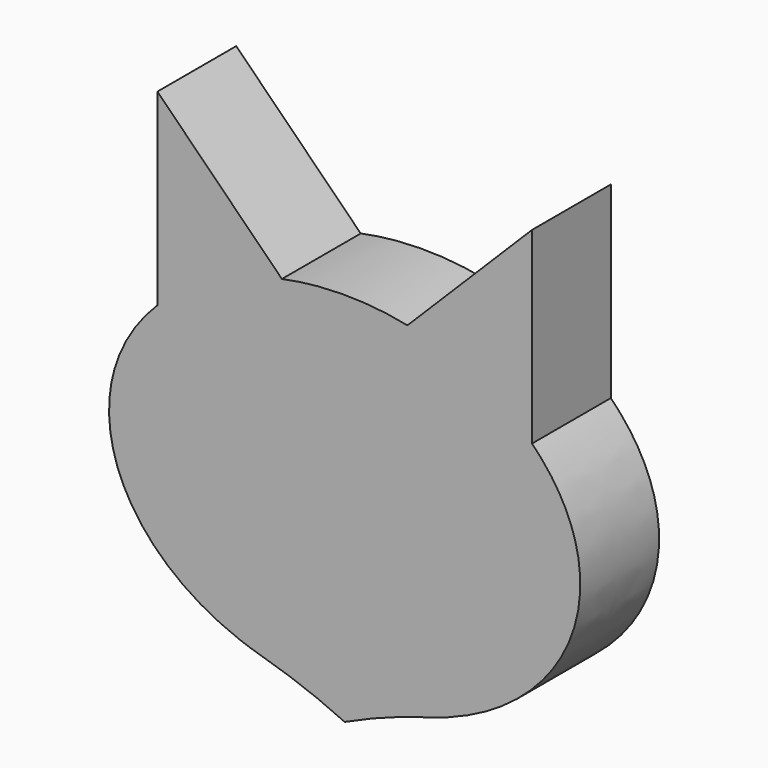
from build123d import *

# Parameters (mm, degrees)
F1_DEPTH    = 25.4
F2_T1_DEPTH = 25.4


# Not quite as in the source:
# - a fillet or chamfer that OpenCascade refuses, or shapes differently, is made with other operations: its cross-section is extruded or revolved along the edge and cut away or added


with BuildPart() as f1:
    # F0 (on Front) → F1 (new body)
    with BuildSketch(Plane.XZ):
        with BuildLine():
            Line((5.7879454147, -45.7212891166), (48.2777159909, 27.8731523232))
            Line((48.2777159909, 27.8731523232), (-48.2777159909, 27.8731523232))
            Line((-48.2777159909, 27.8731523232), (-5.7879454147, -45.7212891166))
            add(Edge.make_bspline(
                [(-5.7879454147, -45.7212891166), (0, -46.1402392948), (5.7879454147, -45.7212891166)],
                knots=[4.6169555149, 4.6169555149, 4.6169555149, 4.8078224459, 4.8078224459, 4.8078224459], degree=2, weights=[1, 0.9954496819, 1]))
        make_face()
        with BuildLine():
            Line((-5.7879454147, -45.7212891166), (-48.2777159909, 27.8731523232))
            add(Edge.make_bspline(
                [(-48.2777159909, 27.8731523232), (-109.7072560683, -32.9641410321), (-9.810773421, -45.327213485)],
                knots=[2.489491462, 2.489491462, 2.489491462, 4.5501606403, 4.5501606403, 4.5501606403], degree=2, weights=[1, 0.5145319732, 1]))
            add(Edge.make_bspline(
                [(-9.810773421, -45.327213485), (-7.808065209, -45.575066323), (-5.7879454147, -45.7212891166)],
                knots=[4.5501606403, 4.5501606403, 4.5501606403, 4.6169555149, 4.6169555149, 4.6169555149], degree=2, weights=[1, 0.9994423574, 1]))
        make_face()
        with BuildLine():
            Line((-48.2777159909, 27.8731523232), (48.2777159909, 27.8731523232))
            add(Edge.make_bspline(
                [(48.2777159909, 27.8731523232), (35.8781903029, 40.1531332703), (16.1845055423, 44.2698445856)],
                knots=[0.6521011916, 0.6521011916, 0.6521011916, 1.3010879793, 1.3010879793, 1.3010879793], degree=2, weights=[1, 0.9478123686, 1]))
            add(Edge.make_bspline(
                [(16.1845055423, 44.2698445856), (0, 47.6530071531), (-16.1845055423, 44.2698445856)],
                knots=[1.3010879793, 1.3010879793, 1.3010879793, 1.8405046743, 1.8405046743, 1.8405046743], degree=2, weights=[1, 0.9638486483, 1]))
            add(Edge.make_bspline(
                [(-16.1845055423, 44.2698445856), (-35.8781903029, 40.1531332703), (-48.2777159909, 27.8731523232)],
                knots=[1.8405046743, 1.8405046743, 1.8405046743, 2.489491462, 2.489491462, 2.489491462], degree=2, weights=[1, 0.9478123686, 1]))
        make_face()
        with BuildLine():
            add(Edge.make_bspline(
                [(9.810773421, -45.327213485), (60.741170722, -39.0241267776), (60.741170722, 0)],
                knots=[4.8746173204, 4.8746173204, 4.8746173204, 6.2831853072, 6.2831853072, 6.2831853072], degree=2, weights=[1, 0.762075353, 1]))
            add(Edge.make_bspline(
                [(60.741170722, 0), (60.741170722, 15.5298586774), (48.2777159909, 27.8731523232)],
                knots=[0, 0, 0, 0.6521011916, 0.6521011916, 0.6521011916], degree=2, weights=[1, 0.947314739, 1]))
            Line((48.2777159909, 27.8731523232), (5.7879454147, -45.7212891166))
            add(Edge.make_bspline(
                [(5.7879454147, -45.7212891166), (7.808065209, -45.575066323), (9.810773421, -45.327213485)],
                knots=[4.8078224459, 4.8078224459, 4.8078224459, 4.8746173204, 4.8746173204, 4.8746173204], degree=2, weights=[1, 0.9994423574, 1]))
        make_face()
        with BuildLine():
            add(Edge.make_bspline(
                [(48.2777159909, 27.8731523232), (35.8781903029, 40.1531332703), (16.1845055423, 44.2698445856)],
                knots=[0.6521011916, 0.6521011916, 0.6521011916, 1.3010879793, 1.3010879793, 1.3010879793], degree=2, weights=[1, 0.9478123686, 1]))
            Line((48.2777159909, 27.8731523232), (48.2777159909, 76.3630550342))
            Line((48.2777159909, 76.3630550342), (16.1845055423, 44.2698445856))
        make_face()
        with BuildLine():
            Line((-48.2777159909, 76.3630550342), (-48.2777159909, 27.8731523232))
            add(Edge.make_bspline(
                [(-16.1845055423, 44.2698445856), (-35.8781903029, 40.1531332703), (-48.2777159909, 27.8731523232)],
                knots=[1.8405046743, 1.8405046743, 1.8405046743, 2.489491462, 2.489491462, 2.489491462], degree=2, weights=[1, 0.9478123686, 1]))
            Line((-16.1845055423, 44.2698445856), (-48.2777159909, 76.3630550342))
        make_face()
        with BuildLine():
            Line((4.1178109195, -48.6140469177), (5.7879454147, -45.7212891166))
            add(Edge.make_bspline(
                [(-5.7879454147, -45.7212891166), (0, -46.1402392948), (5.7879454147, -45.7212891166)],
                knots=[4.6169555149, 4.6169555149, 4.6169555149, 4.8078224459, 4.8078224459, 4.8078224459], degree=2, weights=[1, 0.9954496819, 1]))
            Line((-5.7879454147, -45.7212891166), (-4.1178109195, -48.6140469177))
            Line((-4.1178109195, -48.6140469177), (0, -50.9914661606))
            Line((0, -50.9914661606), (4.1178109195, -48.6140469177))
        make_face()
        with BuildLine():
            add(Edge.make_bspline(
                [(-9.810773421, -45.327213485), (-7.808065209, -45.575066323), (-5.7879454147, -45.7212891166)],
                knots=[4.5501606403, 4.5501606403, 4.5501606403, 4.6169555149, 4.6169555149, 4.6169555149], degree=2, weights=[1, 0.9994423574, 1]))
            Line((-9.810773421, -45.327213485), (-4.1178109195, -48.6140469177))
            Line((-4.1178109195, -48.6140469177), (-5.7879454147, -45.7212891166))
        make_face()
        with BuildLine():
            Line((4.1178109195, -48.6140469177), (9.810773421, -45.327213485))
            add(Edge.make_bspline(
                [(5.7879454147, -45.7212891166), (7.808065209, -45.575066323), (9.810773421, -45.327213485)],
                knots=[4.8078224459, 4.8078224459, 4.8078224459, 4.8746173204, 4.8746173204, 4.8746173204], degree=2, weights=[1, 0.9994423574, 1]))
            Line((5.7879454147, -45.7212891166), (4.1178109195, -48.6140469177))
        make_face()
    extrude(amount=F1_DEPTH)

    # F2: fillet of radius 142.6504443884 on 2 edges, made by hand

    # F2_s2 → F2_t1 (join)
    with BuildSketch(Plane.XZ):
        with BuildLine():
            ThreePointArc((-21.4235280397, -42.9786100328), (-10.5509045607, -46.554957102), (0, -50.9914661606))
            Line((0, -50.9914661606), (1.2104831944, -48.40798205))
            ThreePointArc((1.2104831944, -48.40798205), (-3.4788822666, -45.6885616488), (-8.3842689771, -42.856435311))
            Line((-8.3842689771, -42.856435311), (-9.4603616605, -42.4958054763))
            ThreePointArc((-9.4603616605, -42.4958054763), (-15.0980189089, -41.5804647318), (-20.6415154061, -40.2348687996))
            Line((-20.6415154061, -40.2348687996), (-21.4235280397, -42.9786100328))
        make_face()
        with BuildLine():
            ThreePointArc((0, -50.9914661606), (10.5509045607, -46.554957102), (21.4235280397, -42.9786100328))
            Line((21.4235280397, -42.9786100328), (20.6415154061, -40.2348687996))
            ThreePointArc((20.6415154061, -40.2348687996), (15.0980189089, -41.5804647318), (9.4603616605, -42.4958054763))
            Line((9.4603616605, -42.4958054763), (8.3842689771, -42.856435311))
            ThreePointArc((8.3842689771, -42.856435311), (3.4788822666, -45.6885616488), (-1.2104831944, -48.40798205))
            Line((-1.2104831944, -48.40798205), (0, -50.9914661606))
        make_face()
    extrude(amount=F2_T1_DEPTH)


solid = f1.part
